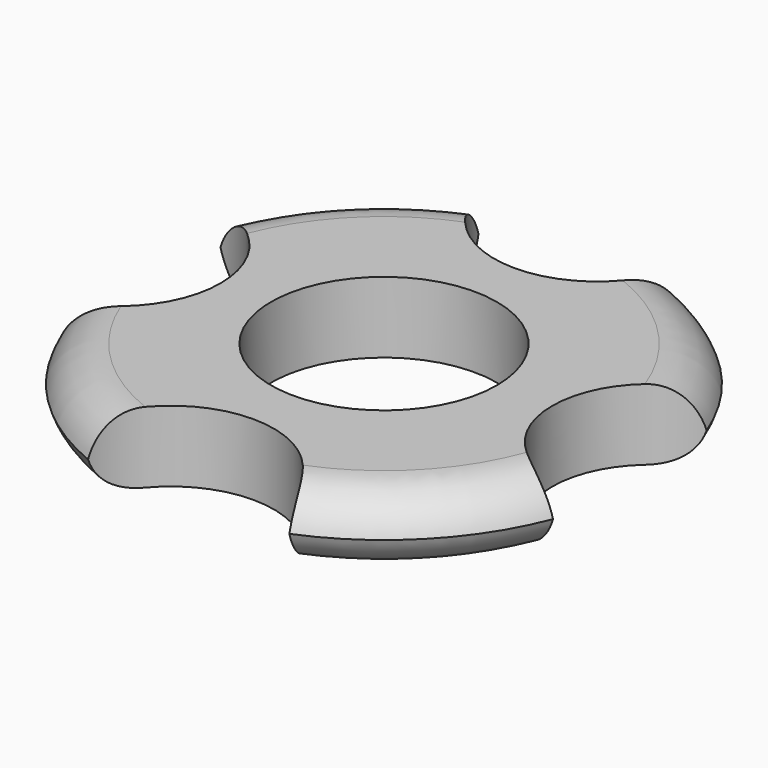
from build123d import *

# Parameters (mm, degrees)
F0_R         = 26.25
F1_DEPTH     = 7
F2_R         = 11.125
F3_DEPTH     = 25.4
F4_R         = 10.16
F4_R_2       = 9.6723514766
F5_DEPTH     = 25.4
F6_T2_ANGLE  = 101.8963155292
F6_T4_ANGLE  = 100.8121389037
F6_T6_ANGLE  = 100.8121389037
F6_T8_ANGLE  = 100.8121389037
F6_T10_ANGLE = 100.8121389037
F6_T12_ANGLE = 101.8963155292
F6_T14_ANGLE = 101.8963155292
F6_T16_ANGLE = 101.8963155292


# Not quite as in the source:
# - a fillet or chamfer that OpenCascade refuses, or shapes differently, is made with other operations: its cross-section is extruded or revolved along the edge and cut away or added


with BuildPart() as f1:
    # F0 (on Top) → F1 (new body)
    with BuildSketch(Plane.XY):
        Circle(F0_R)
    extrude(amount=F1_DEPTH)

    # F2 (on face) → F3 (cut)
    with BuildSketch(Plane.XY.offset(7)):
        Circle(F2_R)
    extrude(amount=-F3_DEPTH, mode=Mode.SUBTRACT)

    # F4 (on face) → F5 (cut)
    with BuildSketch(Plane.XY.offset(7)):
        with Locations((0, -26.25)):
            Circle(F4_R)
        with Locations((-26.25, 0)):
            Circle(F4_R)
        with Locations((0, 26.25)):
            Circle(F4_R)
        with Locations((26.25, 0)):
            Circle(F4_R_2)
    extrude(amount=-F5_DEPTH, mode=Mode.SUBTRACT)

    # F6: fillet of radius 5.08 on 8 edges, made by hand

    # F6_s1 → F6_t2 (revolve, cut)
    with BuildSketch(Plane(origin=(0, 0, 0), x_dir=(0, 0, 1), z_dir=(-0.995551765, 0.0942161515, 0))):
        with BuildLine():
            ThreePointArc((5.08, -26.25), (1.4878975516, -24.7621024484), (0, -21.17))
            Line((0, -21.17), (0, -26.25))
            Line((0, -26.25), (5.08, -26.25))
        make_face()
    revolve(axis=Axis((0, 0, 0), (0, 0, 1)), revolution_arc=F6_T2_ANGLE, mode=Mode.SUBTRACT)

    # F6_s3 → F6_t4 (revolve, cut)
    with BuildSketch(Plane(origin=(0, 0, 0), x_dir=(0, 0, 1), z_dir=(0.0942137746, 0.9955519899, 0))):
        with BuildLine():
            ThreePointArc((5.08, -26.25), (1.4878975516, -24.7621024484), (0, -21.17))
            Line((0, -21.17), (0, -26.25))
            Line((0, -26.25), (5.08, -26.25))
        make_face()
    revolve(axis=Axis((0, 0, 0), (0, 0, 1)), revolution_arc=F6_T4_ANGLE, mode=Mode.SUBTRACT)

    # F6_s5 → F6_t6 (revolve, cut)
    with BuildSketch(Plane(origin=(0, 0, 0), x_dir=(0, 0, 1), z_dir=(0.9955519899, -0.0942137746, 0))):
        with BuildLine():
            ThreePointArc((5.08, -26.25), (1.4878975516, -24.7621024484), (0, -21.17))
            Line((0, -21.17), (0, -26.25))
            Line((0, -26.25), (5.08, -26.25))
        make_face()
    revolve(axis=Axis((0, 0, 0), (0, 0, 1)), revolution_arc=F6_T6_ANGLE, mode=Mode.SUBTRACT)

    # F6_s7 → F6_t8 (revolve, cut)
    with BuildSketch(Plane(origin=(0, 0, 0), x_dir=(0, 0, 1), z_dir=(0.9955519899, -0.0942137746, 0))):
        with BuildLine():
            ThreePointArc((1.92, -26.25), (5.5121024484, -24.7621024484), (7, -21.17))
            Line((7, -21.17), (7, -26.25))
            Line((7, -26.25), (1.92, -26.25))
        make_face()
    revolve(axis=Axis((0, 0, 7), (0, 0, 1)), revolution_arc=F6_T8_ANGLE, mode=Mode.SUBTRACT)

    # F6_s9 → F6_t10 (revolve, cut)
    with BuildSketch(Plane(origin=(0, 0, 0), x_dir=(0, 0, 1), z_dir=(0.0942137746, 0.9955519899, 0))):
        with BuildLine():
            ThreePointArc((1.92, -26.25), (5.5121024484, -24.7621024484), (7, -21.17))
            Line((7, -21.17), (7, -26.25))
            Line((7, -26.25), (1.92, -26.25))
        make_face()
    revolve(axis=Axis((0, 0, 7), (0, 0, 1)), revolution_arc=F6_T10_ANGLE, mode=Mode.SUBTRACT)

    # F6_s11 → F6_t12 (revolve, cut)
    with BuildSketch(Plane(origin=(0, 0, 0), x_dir=(0, 0, 1), z_dir=(-0.995551765, 0.0942161515, 0))):
        with BuildLine():
            ThreePointArc((1.92, -26.25), (5.5121024484, -24.7621024484), (7, -21.17))
            Line((7, -21.17), (7, -26.25))
            Line((7, -26.25), (1.92, -26.25))
        make_face()
    revolve(axis=Axis((0, 0, 7), (0, 0, 1)), revolution_arc=F6_T12_ANGLE, mode=Mode.SUBTRACT)

    # F6_s13 → F6_t14 (revolve, cut)
    with BuildSketch(Plane(origin=(0, 0, 0), x_dir=(0, 0, 1), z_dir=(-0.1130316961, -0.9935913826, 0))):
        with BuildLine():
            ThreePointArc((1.92, -26.25), (5.5121024484, -24.7621024484), (7, -21.17))
            Line((7, -21.17), (7, -26.25))
            Line((7, -26.25), (1.92, -26.25))
        make_face()
    revolve(axis=Axis((0, 0, 7), (0, 0, 1)), revolution_arc=F6_T14_ANGLE, mode=Mode.SUBTRACT)

    # F6_s15 → F6_t16 (revolve, cut)
    with BuildSketch(Plane(origin=(0, 0, 0), x_dir=(0, 0, 1), z_dir=(-0.1130316961, -0.9935913826, 0))):
        with BuildLine():
            ThreePointArc((5.08, -26.25), (1.4878975516, -24.7621024484), (0, -21.17))
            Line((0, -21.17), (0, -26.25))
            Line((0, -26.25), (5.08, -26.25))
        make_face()
    revolve(axis=Axis((0, 0, 0), (0, 0, 1)), revolution_arc=F6_T16_ANGLE, mode=Mode.SUBTRACT)


solid = f1.part
